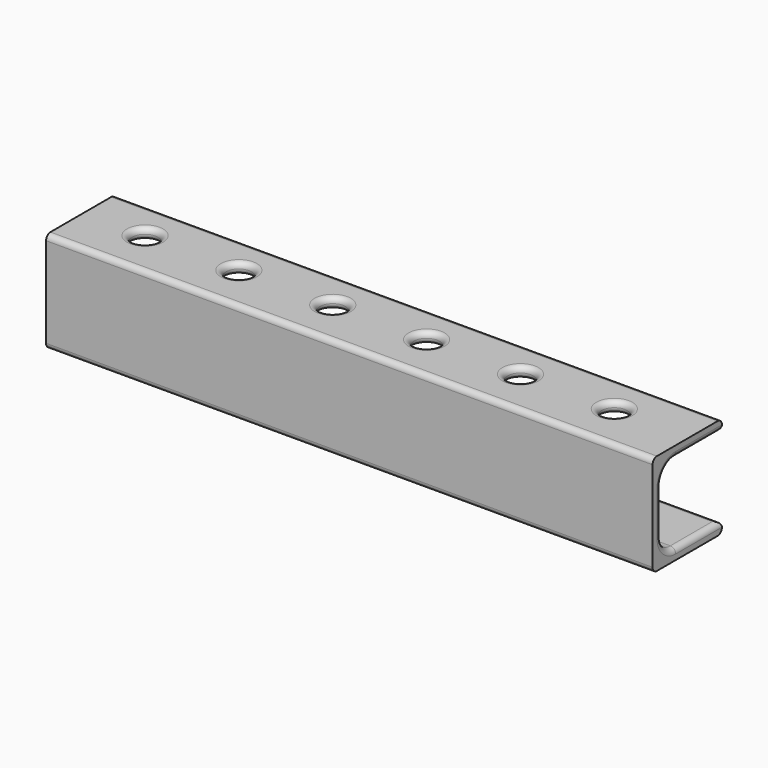
from build123d import *

# Parameters (mm, degrees)
F1_DEPTH = 168
F2_R     = 3.5
F3_DEPTH = 55
F4_R     = 5
F5_R     = 1.49999


# Not quite as in the source:
# - a fillet or chamfer is up to 0.001 mm smaller than in the source, because OpenCascade refuses the exact size


with BuildPart() as f1:
    # F0 (on Right) → F1 (new body)
    with BuildSketch(Plane.YZ):
        Polygon((-24, 0), (0, 0), (0, 3), (-21, 3), (-21, 25), (0, 25), (0, 28), (-24, 28), align=None)
    extrude(amount=F1_DEPTH)

    # F2 (on face) → F3 (cut)
    with BuildSketch(Plane.XY.offset(28)):
        with Locations((17, -11)):
            Circle(F2_R)
        with Locations((43, -11)):
            Circle(F2_R)
        with Locations((69, -11)):
            Circle(F2_R)
        with Locations((95, -11)):
            Circle(F2_R)
        with Locations((121, -11)):
            Circle(F2_R)
        with Locations((147, -11)):
            Circle(F2_R)
    extrude(amount=-F3_DEPTH, mode=Mode.SUBTRACT)

    # F4
    f4_edges = [f1.edges().sort_by_distance(p)[0] for p in [
        (84, -21, 3),
        (84, -21, 25),
    ]]
    fillet(f4_edges, radius=F4_R)

    # F5 (radius 1.5 in the source; OpenCascade refuses exactly that, so slightly less here)
    f5_edges = [f1.edges().sort_by_distance(p)[0] for p in [
        (84, 0, 3),
        (84, 0, 0),
        (84, 0, 28),
        (84, 0, 25),
        (84, -24, 28),
        (84, -24, 0),
        (39.5, -11, 0),
        (13.5, -11, 0),
        (65.5, -11, 0),
        (91.5, -11, 0),
        (117.5, -11, 0),
        (143.5, -11, 0),
        (117.5, -11, 25),
        (91.5, -11, 25),
        (65.5, -11, 25),
        (39.5, -11, 25),
        (0, -8, 25),
        (84, -16, 25),
        (168, -8, 25),
        (143.5, -11, 25),
        (13.5, -11, 25),
        (13.5, -11, 3),
        (39.5, -11, 3),
        (65.5, -11, 3),
        (91.5, -11, 3),
        (117.5, -11, 3),
        (143.5, -11, 3),
        (13.5, -11, 28),
        (39.5, -11, 28),
        (65.5, -11, 28),
        (91.5, -11, 28),
        (117.5, -11, 28),
        (143.5, -11, 28),
    ]]
    fillet(f5_edges, radius=F5_R)


solid = f1.part
